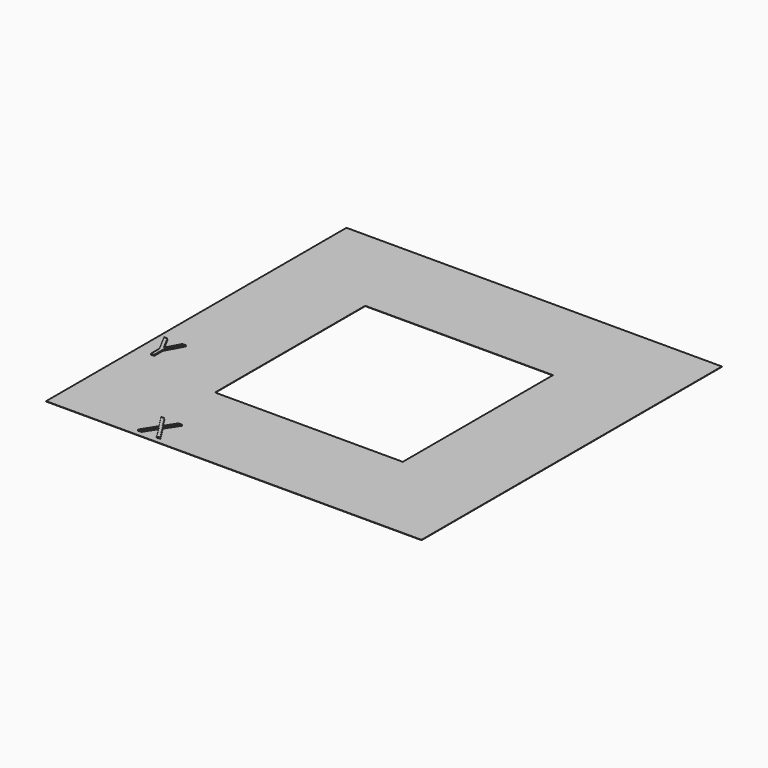
from build123d import *

# Parameters (mm, degrees)
F0_W         = 100
F0_H         = 100
F0_W_2       = 50
F0_H_2       = 50
F1_DEPTH     = 0.0875
F2_TEXT_SIZE = 10.4487666653
F3_DEPTH     = 0.2625


# Not quite as in the source:
# - Text() gives the source's letters only with a copy of the font that has no kerning and outlines rounded to 1/6400 em; it was checked with that copy


with BuildPart() as f1:
    # F0 (on Top) → F1 (new body)
    with BuildSketch(Plane.XY):
        with Locations((14.28270787, -7.3281310499)):
            Rectangle(F0_W, F0_H)
        with Locations((14.28270787, -7.3281310499)):
            Rectangle(F0_W_2, F0_H_2, mode=Mode.SUBTRACT)
    extrude(amount=F1_DEPTH)

    # F2 (on face) → F3 (join)
    with BuildSketch(Plane.XY.offset(0.0875)):
        with Locations((-34.2535031959, -27.3493174464)):
            Text('Y', F2_TEXT_SIZE, font='Open Sans', text_align=(TextAlign.LEFT, TextAlign.BOTTOM))
        with Locations((-12.5331294904, -55.769962776)):
            Text('X', F2_TEXT_SIZE, font='Open Sans', text_align=(TextAlign.LEFT, TextAlign.BOTTOM))
    extrude(amount=F3_DEPTH)


solid = f1.part
